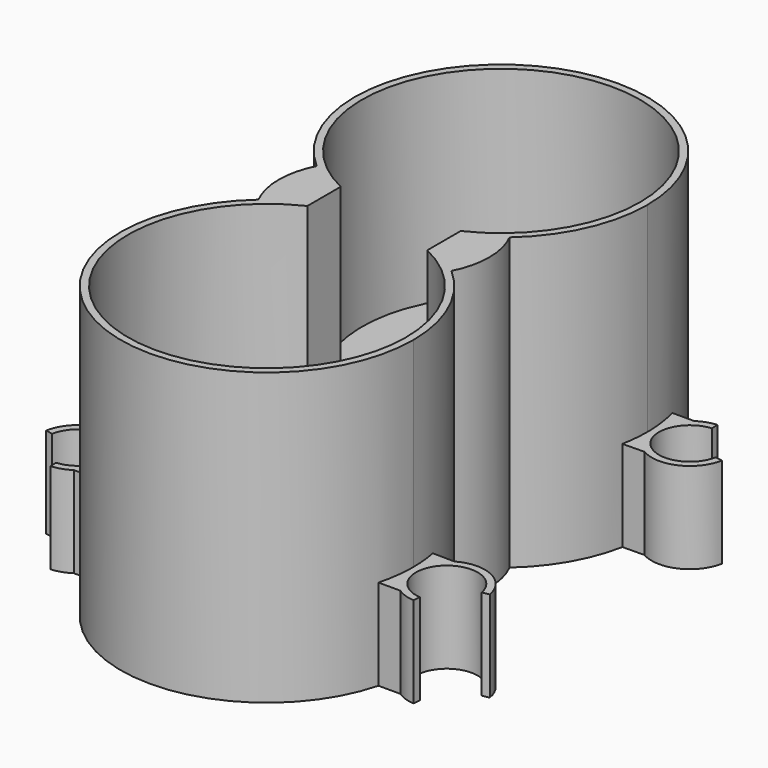
from build123d import *

# Parameters (mm, degrees)
F1_DEPTH = 80
F2_DEPTH = 25
F3_DEPTH = 27
F4_DEPTH = 2
F6_DEPTH = 25


# Not quite as in the source:
# - a feature names something its author has since deleted; it is built from what else it names


with BuildPart() as f1:
    # F0 (on Top) → F1 (new body)
    with BuildSketch(Plane.XY):
        with BuildLine():
            ThreePointArc((-16.5, 5.741848789), (-20.3953119613, 72.6088280072), (38.25, 40.25))
            ThreePointArc((38.25, 40.25), (32.3588280072, 19.8546880387), (16.5, 5.741848789))
            Line((16.5, 5.741848789), (16.5, 3.5374340314))
            ThreePointArc((16.5, 3.5374340314), (17.9795575149, 4.2389182116), (19.4293592277, 5))
            ThreePointArc((19.4293592277, 5), (23.1261233418, 7.306944295), (26.5518360947, 10))
            ThreePointArc((26.5518360947, 10), (36.6658826623, 23.6465199854), (40.25, 40.25))
            ThreePointArc((40.25, 40.25), (-16.6034800146, 76.9158826623), (-26.5518360947, 10))
            ThreePointArc((-26.5518360947, 10), (-23.1261233418, 7.306944295), (-19.4293592277, 5))
            ThreePointArc((-19.4293592277, 5), (-17.9795575149, 4.2389182116), (-16.5, 3.5374340314))
            Line((-16.5, 3.5374340314), (-16.5, 5.741848789))
        make_face()
        with BuildLine():
            Line((-19.4293592277, -5), (-19.4293592277, 5))
            ThreePointArc((-19.4293592277, 5), (-23.1261233418, 7.306944295), (-26.5518360947, 10))
            ThreePointArc((-26.5518360947, 10), (-28.9559181524, 0), (-26.5518360947, -10))
            ThreePointArc((-26.5518360947, -10), (-23.1261233418, -7.306944295), (-19.4293592277, -5))
        make_face()
        with BuildLine():
            Line((-16.5, -5.741848789), (-16.5, -3.5374340314))
            ThreePointArc((-16.5, -3.5374340314), (-17.9795575149, -4.2389182116), (-19.4293592277, -5))
            ThreePointArc((-19.4293592277, -5), (-23.1261233418, -7.306944295), (-26.5518360947, -10))
            ThreePointArc((-26.5518360947, -10), (-16.6034800146, -76.9158826623), (40.25, -40.25))
            ThreePointArc((40.25, -40.25), (36.6658826623, -23.6465199854), (26.5518360947, -10))
            ThreePointArc((26.5518360947, -10), (23.1261233418, -7.306944295), (19.4293592277, -5))
            ThreePointArc((19.4293592277, -5), (17.9795575149, -4.2389182116), (16.5, -3.5374340314))
            Line((16.5, -3.5374340314), (16.5, -5.741848789))
            ThreePointArc((16.5, -5.741848789), (32.3588280072, -19.8546880387), (38.25, -40.25))
            ThreePointArc((38.25, -40.25), (-20.3953119613, -72.6088280072), (-16.5, -5.741848789))
        make_face()
        with BuildLine():
            ThreePointArc((26.5518360947, 10), (23.1261233418, 7.306944295), (19.4293592277, 5))
            Line((19.4293592277, 5), (19.4293592277, -5))
            ThreePointArc((19.4293592277, -5), (23.1261233418, -7.306944295), (26.5518360947, -10))
            ThreePointArc((26.5518360947, -10), (28.9559181524, 0), (26.5518360947, 10))
        make_face()
        with BuildLine():
            ThreePointArc((19.4293592277, 5), (17.9795575149, 4.2389182116), (16.5, 3.5374340314))
            Line((16.5, 3.5374340314), (16.5, -3.5374340314))
            ThreePointArc((16.5, -3.5374340314), (17.9795575149, -4.2389182116), (19.4293592277, -5))
            Line((19.4293592277, -5), (19.4293592277, 5))
        make_face()
        with BuildLine():
            Line((-16.5, -3.5374340314), (-16.5, 3.5374340314))
            ThreePointArc((-16.5, 3.5374340314), (-17.9795575149, 4.2389182116), (-19.4293592277, 5))
            Line((-19.4293592277, 5), (-19.4293592277, -5))
            ThreePointArc((-19.4293592277, -5), (-17.9795575149, -4.2389182116), (-16.5, -3.5374340314))
        make_face()
    extrude(amount=F1_DEPTH)

    # F0 (on Top) → F2 (join)
    with BuildSketch(Plane.XY):
        with BuildLine():
            Line((-16.5, -50), (-16.5, -5.741848789))
            ThreePointArc((-16.5, -5.741848789), (-20.3953119613, -72.6088280072), (38.25, -40.25))
            ThreePointArc((38.25, -40.25), (32.3588280072, -19.8546880387), (16.5, -5.741848789))
            Line((16.5, -5.741848789), (16.5, -50))
            Line((16.5, -50), (-16.5, -50))
        make_face()
        with BuildLine():
            ThreePointArc((16.5, 5.741848789), (32.3588280072, 19.8546880387), (38.25, 40.25))
            ThreePointArc((38.25, 40.25), (-20.3953119613, 72.6088280072), (-16.5, 5.741848789))
            Line((-16.5, 5.741848789), (-16.5, 50))
            Line((-16.5, 50), (16.5, 50))
            Line((16.5, 50), (16.5, 5.741848789))
        make_face()
        with BuildLine():
            ThreePointArc((16.5, -5.741848789), (0, -2), (-16.5, -5.741848789))
            Line((-16.5, -5.741848789), (-16.5, -50))
            Line((-16.5, -50), (16.5, -50))
            Line((16.5, -50), (16.5, -5.741848789))
        make_face()
        with BuildLine():
            Line((-16.5, 50), (-16.5, 5.741848789))
            ThreePointArc((-16.5, 5.741848789), (0, 2), (16.5, 5.741848789))
            Line((16.5, 5.741848789), (16.5, 50))
            Line((16.5, 50), (-16.5, 50))
        make_face()
        with BuildLine():
            ThreePointArc((19.4293592277, 5), (17.9795575149, 4.2389182116), (16.5, 3.5374340314))
            Line((16.5, 3.5374340314), (16.5, -3.5374340314))
            ThreePointArc((16.5, -3.5374340314), (17.9795575149, -4.2389182116), (19.4293592277, -5))
            Line((19.4293592277, -5), (19.4293592277, 5))
        make_face()
        with BuildLine():
            Line((-16.5, -3.5374340314), (-16.5, 3.5374340314))
            ThreePointArc((-16.5, 3.5374340314), (-17.9795575149, 4.2389182116), (-19.4293592277, 5))
            Line((-19.4293592277, 5), (-19.4293592277, -5))
            ThreePointArc((-19.4293592277, -5), (-17.9795575149, -4.2389182116), (-16.5, -3.5374340314))
        make_face()
        with BuildLine():
            ThreePointArc((1.604e-07, 0), (-8.4374675441, 0.8942934069), (-16.5, 3.5374340314))
            Line((-16.5, 3.5374340314), (-16.5, -3.5374340314))
            ThreePointArc((-16.5, -3.5374340314), (-8.4374675441, -0.8942934069), (1.604e-07, 0))
        make_face()
        with BuildLine():
            ThreePointArc((16.5, 5.741848789), (0, 2), (-16.5, 5.741848789))
            Line((-16.5, 5.741848789), (-16.5, 3.5374340314))
            ThreePointArc((-16.5, 3.5374340314), (-8.4374675441, 0.8942934069), (1.604e-07, 0))
            ThreePointArc((1.604e-07, 0), (8.437467701, 0.8942934405), (16.5, 3.5374340314))
            Line((16.5, 3.5374340314), (16.5, 5.741848789))
        make_face()
        with BuildLine():
            ThreePointArc((16.5, -3.5374340314), (8.437467701, -0.8942934405), (1.604e-07, 0))
            ThreePointArc((1.604e-07, 0), (-8.4374675441, -0.8942934069), (-16.5, -3.5374340314))
            Line((-16.5, -3.5374340314), (-16.5, -5.741848789))
            ThreePointArc((-16.5, -5.741848789), (0, -2), (16.5, -5.741848789))
            Line((16.5, -5.741848789), (16.5, -3.5374340314))
        make_face()
        with BuildLine():
            Line((16.5, -3.5374340314), (16.5, 3.5374340314))
            ThreePointArc((16.5, 3.5374340314), (8.437467701, 0.8942934405), (1.604e-07, 0))
            ThreePointArc((1.604e-07, 0), (8.437467701, -0.8942934405), (16.5, -3.5374340314))
        make_face()
    extrude(amount=F2_DEPTH)

    # F0 (on Top) → F3 (cut)
    with BuildSketch(Plane.XY):
        with BuildLine():
            Line((-16.5, 50), (-16.5, 5.741848789))
            ThreePointArc((-16.5, 5.741848789), (0, 2), (16.5, 5.741848789))
            Line((16.5, 5.741848789), (16.5, 50))
            Line((16.5, 50), (-16.5, 50))
        make_face()
        with BuildLine():
            ThreePointArc((16.5, -5.741848789), (0, -2), (-16.5, -5.741848789))
            Line((-16.5, -5.741848789), (-16.5, -50))
            Line((-16.5, -50), (16.5, -50))
            Line((16.5, -50), (16.5, -5.741848789))
        make_face()
        with BuildLine():
            ThreePointArc((16.5, 5.741848789), (0, 2), (-16.5, 5.741848789))
            Line((-16.5, 5.741848789), (-16.5, 3.5374340314))
            ThreePointArc((-16.5, 3.5374340314), (-8.4374675441, 0.8942934069), (1.604e-07, 0))
            ThreePointArc((1.604e-07, 0), (8.437467701, 0.8942934405), (16.5, 3.5374340314))
            Line((16.5, 3.5374340314), (16.5, 5.741848789))
        make_face()
        with BuildLine():
            ThreePointArc((16.5, -3.5374340314), (8.437467701, -0.8942934405), (1.604e-07, 0))
            ThreePointArc((1.604e-07, 0), (-8.4374675441, -0.8942934069), (-16.5, -3.5374340314))
            Line((-16.5, -3.5374340314), (-16.5, -5.741848789))
            ThreePointArc((-16.5, -5.741848789), (0, -2), (16.5, -5.741848789))
            Line((16.5, -5.741848789), (16.5, -3.5374340314))
        make_face()
        with BuildLine():
            Line((16.5, -3.5374340314), (16.5, 3.5374340314))
            ThreePointArc((16.5, 3.5374340314), (8.437467701, 0.8942934405), (1.604e-07, 0))
            ThreePointArc((1.604e-07, 0), (8.437467701, -0.8942934405), (16.5, -3.5374340314))
        make_face()
        with BuildLine():
            ThreePointArc((1.604e-07, 0), (-8.4374675441, 0.8942934069), (-16.5, 3.5374340314))
            Line((-16.5, 3.5374340314), (-16.5, -3.5374340314))
            ThreePointArc((-16.5, -3.5374340314), (-8.4374675441, -0.8942934069), (1.604e-07, 0))
        make_face()
    extrude(amount=F3_DEPTH, mode=Mode.SUBTRACT)

    # F0 (on Top) → F4 (join)
    with BuildSketch(Plane.XY):
        with BuildLine():
            ThreePointArc((16.5, -5.741848789), (0, -2), (-16.5, -5.741848789))
            Line((-16.5, -5.741848789), (-16.5, -50))
            Line((-16.5, -50), (16.5, -50))
            Line((16.5, -50), (16.5, -5.741848789))
        make_face()
        with BuildLine():
            Line((16.5, -3.5374340314), (16.5, 3.5374340314))
            ThreePointArc((16.5, 3.5374340314), (8.437467701, 0.8942934405), (1.604e-07, 0))
            ThreePointArc((1.604e-07, 0), (8.437467701, -0.8942934405), (16.5, -3.5374340314))
        make_face()
        with BuildLine():
            ThreePointArc((16.5, -3.5374340314), (8.437467701, -0.8942934405), (1.604e-07, 0))
            ThreePointArc((1.604e-07, 0), (-8.4374675441, -0.8942934069), (-16.5, -3.5374340314))
            Line((-16.5, -3.5374340314), (-16.5, -5.741848789))
            ThreePointArc((-16.5, -5.741848789), (0, -2), (16.5, -5.741848789))
            Line((16.5, -5.741848789), (16.5, -3.5374340314))
        make_face()
        with BuildLine():
            Line((-16.5, 50), (-16.5, 5.741848789))
            ThreePointArc((-16.5, 5.741848789), (0, 2), (16.5, 5.741848789))
            Line((16.5, 5.741848789), (16.5, 50))
            Line((16.5, 50), (-16.5, 50))
        make_face()
        with BuildLine():
            ThreePointArc((1.604e-07, 0), (-8.4374675441, 0.8942934069), (-16.5, 3.5374340314))
            Line((-16.5, 3.5374340314), (-16.5, -3.5374340314))
            ThreePointArc((-16.5, -3.5374340314), (-8.4374675441, -0.8942934069), (1.604e-07, 0))
        make_face()
        with BuildLine():
            ThreePointArc((16.5, 5.741848789), (0, 2), (-16.5, 5.741848789))
            Line((-16.5, 5.741848789), (-16.5, 3.5374340314))
            ThreePointArc((-16.5, 3.5374340314), (-8.4374675441, 0.8942934069), (1.604e-07, 0))
            ThreePointArc((1.604e-07, 0), (8.437467701, 0.8942934405), (16.5, 3.5374340314))
            Line((16.5, 3.5374340314), (16.5, 5.741848789))
        make_face()
        with BuildLine():
            ThreePointArc((19.4293592277, 5), (17.9795575149, 4.2389182116), (16.5, 3.5374340314))
            Line((16.5, 3.5374340314), (16.5, -3.5374340314))
            ThreePointArc((16.5, -3.5374340314), (17.9795575149, -4.2389182116), (19.4293592277, -5))
            Line((19.4293592277, -5), (19.4293592277, 5))
        make_face()
    extrude(amount=F4_DEPTH)

    # F5 (on Top) → F6 (join)
    with BuildSketch(Plane.XY):
        with BuildLine():
            Line((50.0608983682, 50.276728797), (49.9043477191, 52.2705923566))
            ThreePointArc((49.9043477191, 52.2705923566), (47.2974067112, 51.7271782555), (44.9110131577, 50.5454142725))
            ThreePointArc((44.9110131577, 50.5454142725), (41.3964470277, 46.6199643352), (40.2311547735, 41.4815378976))
            ThreePointArc((40.2311547735, 41.4815378976), (41.7260907127, 36.3947279075), (45.5157965565, 32.6868175855))
            ThreePointArc((45.5157965565, 32.6868175855), (55.1559261055, 32.2829416087), (61.0556229863, 39.9176511802))
            Line((61.0556229863, 39.9176511802), (59.0881212036, 40.276728797))
            ThreePointArc((59.0881212036, 40.276728797), (44.416786122, 36.1071252956), (50.0608983682, 50.276728797))
        make_face()
        with BuildLine():
            ThreePointArc((45.5157965565, 32.6868175855), (41.7260907127, 36.3947279075), (40.2311547735, 41.4815378976))
            ThreePointArc((40.2311547735, 41.4815378976), (40.2452884176, 40.8658410379), (40.25, 40.25))
            ThreePointArc((40.25, 40.25), (40.0661847306, 36.4076906509), (39.5164178318, 32.6004757181))
            Line((39.5164178318, 32.6004757181), (45.5157965565, 32.6868175855))
        make_face()
        with BuildLine():
            ThreePointArc((40.2311547735, 41.4815378976), (41.3964470277, 46.6199643352), (44.9110131577, 50.5454142725))
            Line((44.9110131577, 50.5454142725), (38.9110131577, 50.5454142725))
            ThreePointArc((38.9110131577, 50.5454142725), (39.8297520698, 46.0511507526), (40.2311547735, 41.4815378976))
        make_face()
        with BuildLine():
            ThreePointArc((-40.2311547563, 41.4815384597), (-41.3964471567, 46.619964585), (-44.9110131577, 50.5454142725))
            ThreePointArc((-44.9110131577, 50.5454142725), (-47.2974067112, 51.7271782555), (-49.9043477191, 52.2705923566))
            Line((-49.9043477191, 52.2705923566), (-50.0477133056, 50.2756832334))
            ThreePointArc((-50.0477133056, 50.2756832334), (-44.4212194253, 36.102218097), (-59.0881212036, 40.276728797))
            Line((-59.0881212036, 40.276728797), (-61.0556229863, 39.9176511802))
            ThreePointArc((-61.0556229863, 39.9176511802), (-55.1559261055, 32.2829416087), (-45.5157965565, 32.6868175855))
            ThreePointArc((-45.5157965565, 32.6868175855), (-41.7260905679, 36.3947281485), (-40.2311547563, 41.4815384597))
        make_face()
        with BuildLine():
            ThreePointArc((-39.5164178318, 32.6004757181), (-40.1202835518, 37.021169295), (-40.2311547563, 41.4815384597))
            ThreePointArc((-40.2311547563, 41.4815384597), (-41.7260905679, 36.3947281485), (-45.5157965565, 32.6868175855))
            Line((-45.5157965565, 32.6868175855), (-39.5164178318, 32.6004757181))
        make_face()
        with BuildLine():
            ThreePointArc((-40.2311547563, 41.4815384597), (-39.8297520293, 46.0511510308), (-38.9110131577, 50.5454142725))
            Line((-38.9110131577, 50.5454142725), (-44.9110131577, 50.5454142725))
            ThreePointArc((-44.9110131577, 50.5454142725), (-41.3964471567, 46.619964585), (-40.2311547563, 41.4815384597))
        make_face()
        with BuildLine():
            ThreePointArc((61.0556229863, -39.9176511802), (55.1559261055, -32.2829416087), (45.5157965565, -32.6868175855))
            ThreePointArc((45.5157965565, -32.6868175855), (41.7260905575, -36.3947281657), (40.231154755, -41.4815384999))
            ThreePointArc((40.231154755, -41.4815384999), (41.3964471659, -46.6199646029), (44.9110131577, -50.5454142725))
            ThreePointArc((44.9110131577, -50.5454142725), (47.2974067112, -51.7271782555), (49.9043477191, -52.2705923566))
            Line((49.9043477191, -52.2705923566), (50.0608983682, -50.276728797))
            ThreePointArc((50.0608983682, -50.276728797), (44.416786122, -36.1071252956), (59.0881212036, -40.276728797))
            Line((59.0881212036, -40.276728797), (61.0556229863, -39.9176511802))
        make_face()
        with BuildLine():
            Line((45.5157965565, -32.6868175855), (39.5164178318, -32.6004757181))
            ThreePointArc((39.5164178318, -32.6004757181), (40.0661847306, -36.4076906509), (40.25, -40.25))
            ThreePointArc((40.25, -40.25), (40.245288413, -40.8658413392), (40.231154755, -41.4815384999))
            ThreePointArc((40.231154755, -41.4815384999), (41.7260905575, -36.3947281657), (45.5157965565, -32.6868175855))
        make_face()
        with BuildLine():
            ThreePointArc((44.9110131577, -50.5454142725), (41.3964471659, -46.6199646029), (40.231154755, -41.4815384999))
            ThreePointArc((40.231154755, -41.4815384999), (39.8297520264, -46.0511510507), (38.9110131577, -50.5454142725))
            Line((38.9110131577, -50.5454142725), (44.9110131577, -50.5454142725))
        make_face()
        with BuildLine():
            ThreePointArc((-40.2311547578, -41.481538411), (-40.1202835499, -37.0211692707), (-39.5164178318, -32.6004757181))
            Line((-39.5164178318, -32.6004757181), (-45.5157965565, -32.6868175855))
            ThreePointArc((-45.5157965565, -32.6868175855), (-41.7260905804, -36.3947281276), (-40.2311547578, -41.481538411))
        make_face()
        with BuildLine():
            ThreePointArc((-38.9110131577, -50.5454142725), (-39.8297520328, -46.0511510067), (-40.2311547578, -41.481538411))
            ThreePointArc((-40.2311547578, -41.481538411), (-41.3964471455, -46.6199645634), (-44.9110131577, -50.5454142725))
            Line((-44.9110131577, -50.5454142725), (-38.9110131577, -50.5454142725))
        make_face()
        with BuildLine():
            ThreePointArc((-40.2311547578, -41.481538411), (-41.7260905804, -36.3947281276), (-45.5157965565, -32.6868175855))
            ThreePointArc((-45.5157965565, -32.6868175855), (-55.1559261055, -32.2829416087), (-61.0556229863, -39.9176511802))
            Line((-61.0556229863, -39.9176511802), (-59.0881212036, -40.276728797))
            ThreePointArc((-59.0881212036, -40.276728797), (-44.4212194253, -36.102218097), (-50.0477133056, -50.2756832334))
            Line((-50.0477133056, -50.2756832334), (-49.9043477191, -52.2705923566))
            ThreePointArc((-49.9043477191, -52.2705923566), (-47.2974067112, -51.7271782555), (-44.9110131577, -50.5454142725))
            ThreePointArc((-44.9110131577, -50.5454142725), (-41.3964471455, -46.6199645634), (-40.2311547578, -41.481538411))
        make_face()
    extrude(amount=F6_DEPTH)


solid = f1.part
